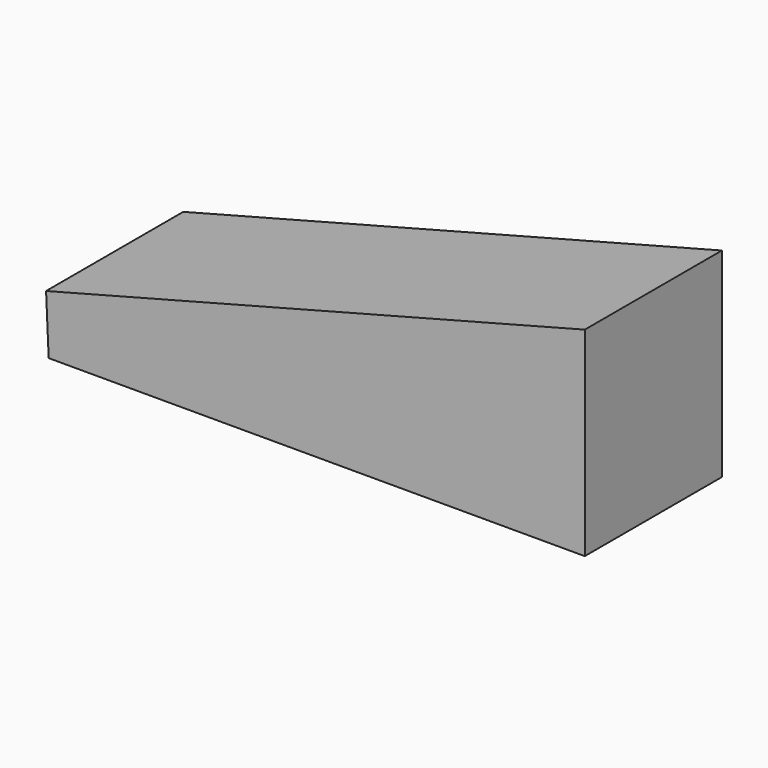
from build123d import *

# Parameters (mm, degrees)
F1_DEPTH = 25.4


# Not quite as in the source:
# - the program builds the solid bodies; features that only make, move or delete a surface that nothing else refers to are left out


with BuildPart() as f1:
    # F0 (on Front) → F1 (new body)
    with BuildSketch(Plane.XZ):
        Polygon((-38.9497131109, 8.63417238), (-38.5659709573, 0), (40.8684201539, 0), (40.8684201539, 29.5480582863), align=None)
    extrude(amount=F1_DEPTH)


solid = f1.part
